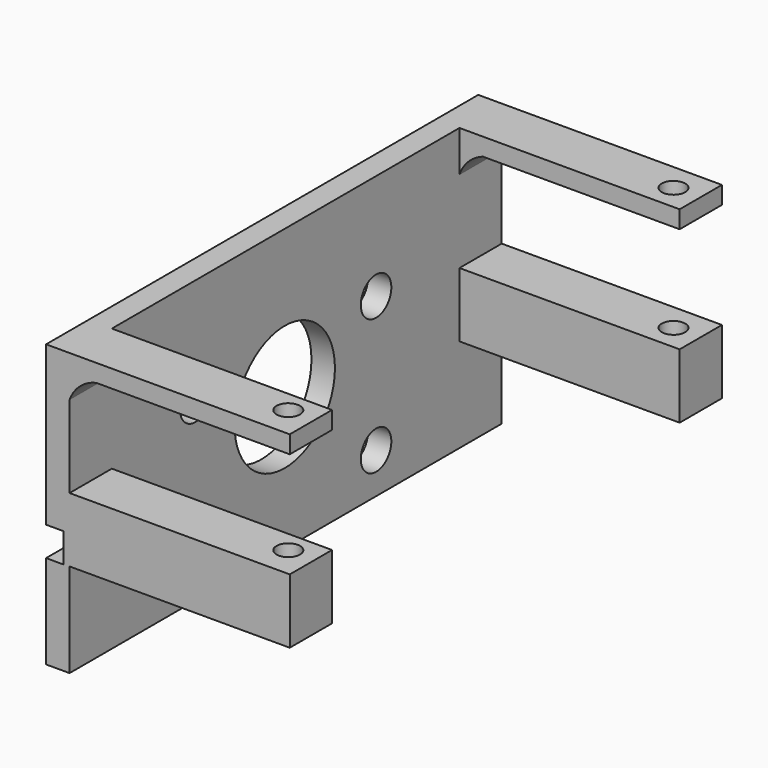
from build123d import *

# Parameters (mm, degrees)
F0_W         = 92
F0_H         = 48
F1_DEPTH     = 4
F2_R         = 3.25
F2_R_2       = 10.6786712851
F3_DEPTH     = 25
F4_W         = 9
F4_H         = 11
F4_H_2       = 3
F5_DEPTH     = 37.5
F6_R         = 2
F7_DEPTH     = 40
F8_W         = 0.1783174183
F8_H         = 5
F8_W_2       = 4.8216825817
F8_W_3       = 5
F9_DEPTH     = 3
F10_T4_DEPTH = 5
F12_DEPTH    = 9
F14_DEPTH    = 9


# Not quite as in the source:
# - a fillet or chamfer that OpenCascade refuses, or shapes differently, is made with other operations: its cross-section is extruded or revolved along the edge and cut away or added


with BuildPart() as f1:
    # F0 (on Right) → F1 (new body)
    with BuildSketch(Plane.YZ):
        with Locations((-47.0313817766, -16.1659868658)):
            Rectangle(F0_W, F0_H)
    extrude(amount=F1_DEPTH)

    # F2 (on face) → F3 (cut)
    with BuildSketch(Plane.YZ.offset(4)):
        with Locations((-66.2813817766, -10.1659868658)):
            Circle(F2_R)
        with Locations((-27.7813817766, -10.1659868658)):
            Circle(F2_R)
        with Locations((-66.2813817766, -33.2659868658)):
            Circle(F2_R)
        with Locations((-27.7813817766, -33.2659868658)):
            Circle(F2_R)
        with Locations((-47.217734158, -17.3795577139)):
            Circle(F2_R_2)
    extrude(amount=-F3_DEPTH, mode=Mode.SUBTRACT)

    # F4 (on face) → F5 (join)
    with BuildSketch(Plane.YZ.offset(4)):
        with Locations((-88.5313817766, -18.6659868658)):
            Rectangle(F4_W, F4_H)
        with Locations((-5.5313817766, -18.6659868658)):
            Rectangle(F4_W, F4_H)
        with Locations((-88.5313817766, 6.3340131342)):
            Rectangle(F4_W, F4_H_2)
        with Locations((-5.5313817766, 6.3340131342)):
            Rectangle(F4_W, F4_H_2)
    extrude(amount=F5_DEPTH)

    # F6 (on face) → F7 (cut)
    with BuildSketch(Plane.XY.offset(7.8340131342)):
        with Locations((37, -5.7174442336)):
            Circle(F6_R)
        with Locations((37, -87.7174442336)):
            Circle(F6_R)
    extrude(amount=-F7_DEPTH, mode=Mode.SUBTRACT)

    # F8 (on face) → F9 (cut)
    with BuildSketch(Plane(origin=(0, 0, 0), x_dir=(0, -1, 0), z_dir=(-1, 0, 0))):
        with Locations((0.9422230674, -21.7159868658)):
            Rectangle(F8_W, F8_H)
        with Locations((3.4422230674, -21.7159868658)):
            Rectangle(F8_W_2, F8_H)
        with Locations((90.5313817766, -21.7159868658)):
            Rectangle(F8_W_3, F8_H)
    extrude(amount=-F9_DEPTH, mode=Mode.SUBTRACT)

    # F10: chamfer of 5 on 1 edges, made by hand


with BuildPart() as f10_tool2:
    # F10_s3 → F10_t4 (new body)
    with BuildSketch(Plane.XY.offset(-19.2159868658)):
        Polygon((8, -1.0313817766), (3, -6.0313817766), (3, -1.0313817766), align=None)
    extrude(amount=-F10_T4_DEPTH)

    split(bisect_by=Plane.XZ.offset(5.8530643582), keep=Keep.BOTTOM)


with BuildPart() as f1_1:
    add(f1.part)

    # F10_t1: cut F10_tool2
    add(f10_tool2.part, mode=Mode.SUBTRACT)

    # F11 (on face) → F12 (join)
    with BuildSketch(Plane(origin=(0, -1.0313817766, 0), x_dir=(-1, 0, 0), z_dir=(0, 1, 0))):
        with BuildLine():
            ThreePointArc((-8, 4.8340131342), (-5.539111548, 3.2949015862), (-4, 0.8340131342))
            Line((-4, 0.8340131342), (-4, 4.8340131342))
            Line((-4, 4.8340131342), (-8, 4.8340131342))
        make_face()
    extrude(amount=-F12_DEPTH)

    # F13 (on face) → F14 (join)
    with BuildSketch(Plane.XZ.offset(93.0313817766)):
        with BuildLine():
            ThreePointArc((4, 0.8340131342), (5.7533122895, 3.408733727), (8.5231261328, 4.8340131342))
            Line((8.5231261328, 4.8340131342), (4, 4.8340131342))
            Line((4, 4.8340131342), (4, 0.8340131342))
        make_face()
    extrude(amount=-F14_DEPTH)


solid = f1_1.part
